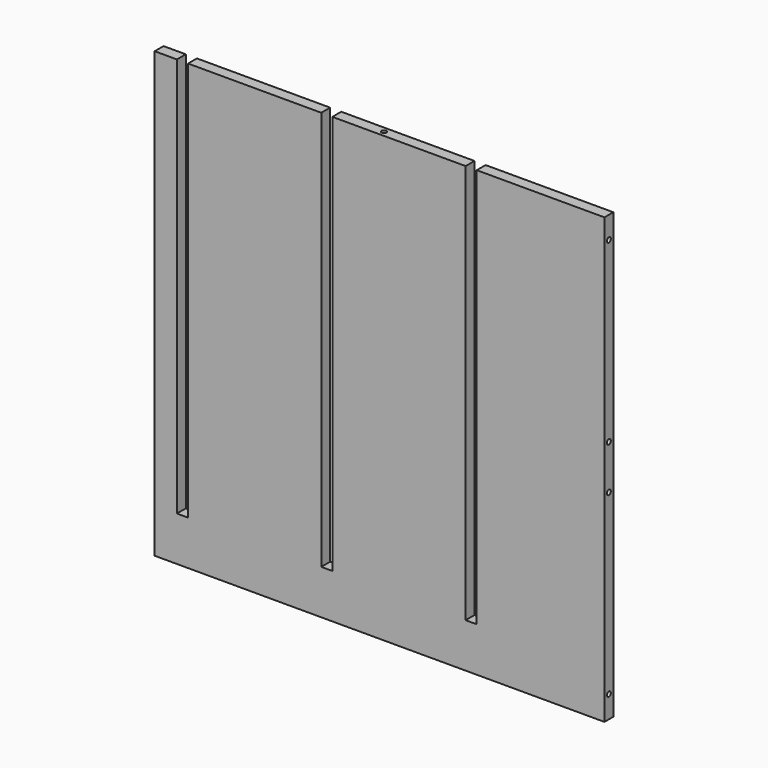
from build123d import *

# Parameters (mm, degrees)
F1_DEPTH       = 5
F6_D           = 4.4
F6_DEPTH       = 12
F6_TIP         = 1.3218933619
F7_D           = 4.4
F7_DEPTH       = 12
F7_TIP         = 1.3218933619
F7_ON_F4_D     = 4.4
F7_ON_F4_DEPTH = 12
F7_ON_F4_TIP   = 1.3218933619
F7_ON_F5_D     = 4.4
F7_ON_F5_DEPTH = 12
F7_ON_F5_TIP   = 1.3218933619


# Not quite as in the source:
# - a feature names something its author has since deleted; it is built from what else it names


with BuildPart() as f1:
    # F0 (on Front) → F1 (new body, symmetric)
    with BuildSketch(Plane.XZ):
        Polygon((-202.5, -200), (202.5, -200), (202.5, 200), (87.5, 200), (87.5, -160), (77.5, -160), (77.5, 200), (-42.5, 200), (-42.5, -160), (-52.5, -160), (-52.5, 200), (-172.5, 200), (-172.5, -160), (-182.5, -160), (-182.5, 200), (-202.5, 200), align=None)
    extrude(amount=F1_DEPTH, both=True)

    # F6
    with Locations(Plane.XY.offset(200)):
        with Locations((0, 0)):
            Hole(F6_D / 2, depth=F6_DEPTH)
            with Locations((0, 0, -(F6_DEPTH + F6_TIP / 2))):  # 118° drill point
                Cone(0, F6_D / 2, F6_TIP, mode=Mode.SUBTRACT)

    # F7
    with Locations(Plane(origin=(-202.5, 0, 0), x_dir=(0, -1, 0), z_dir=(-1, 0, 0))):
        with Locations((0, -180), (0, -20), (0, 20), (0, 180)):
            Hole(F7_D / 2, depth=F7_DEPTH)
            with Locations((0, 0, -(F7_DEPTH + F7_TIP / 2))):  # 118° drill point
                Cone(0, F7_D / 2, F7_TIP, mode=Mode.SUBTRACT)

    # F7 on F4
    with Locations(Plane.YZ.offset(202.5)):
        with Locations((0, -180), (0, -20), (0, 180), (0, 20)):
            Hole(F7_ON_F4_D / 2, depth=F7_ON_F4_DEPTH)
            with Locations((0, 0, -(F7_ON_F4_DEPTH + F7_ON_F4_TIP / 2))):  # 118° drill point
                Cone(0, F7_ON_F4_D / 2, F7_ON_F4_TIP, mode=Mode.SUBTRACT)

    # F7 on F5
    with Locations(Plane(origin=(0, 0, -200), x_dir=(1, 0, 0), z_dir=(0, 0, -1))):
        with Locations((-182.5, 0), (-62.5, 0), (62.5, 0), (182.5, 0)):
            Hole(F7_ON_F5_D / 2, depth=F7_ON_F5_DEPTH)
            with Locations((0, 0, -(F7_ON_F5_DEPTH + F7_ON_F5_TIP / 2))):  # 118° drill point
                Cone(0, F7_ON_F5_D / 2, F7_ON_F5_TIP, mode=Mode.SUBTRACT)


solid = f1.part
